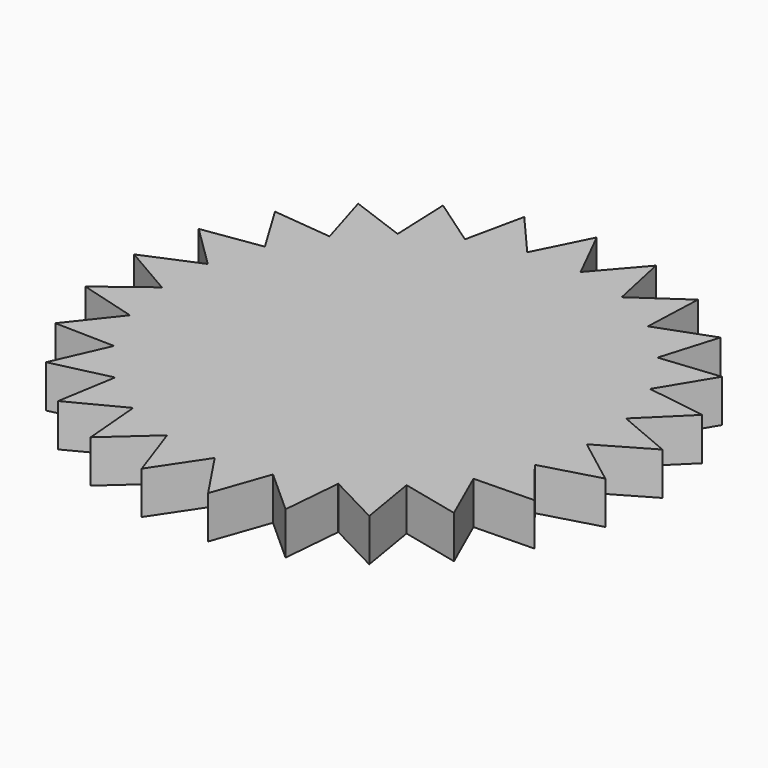
from build123d import *

# Parameters (mm, degrees)
F0_R            = 63.5
F1_DEPTH        = 6.35
F3_DEPTH        = 12.7
F3_COPIES_COUNT = 25


# Not quite as in the source:
# - a pattern or mirror of a feature is missing from the dataset's text; its kind, count and spacing are read off the source's solid


with BuildPart() as f1:
    # F0 (on Top) → F1 (new body, symmetric)
    with BuildSketch(Plane.XY):
        Circle(F0_R)
    extrude(amount=F1_DEPTH, both=True)

    # F2 (on face) → F3 (join, through all)
    with BuildSketch(Plane.XY.offset(6.35)):
        with BuildLine():
            Line((0, 78.9130567023), (-7.9355522703, 63.002198455))
            ThreePointArc((-7.9355522703, 63.002198455), (0, 63.5), (7.9355522703, 63.002198455))
            Line((7.9355522703, 63.002198455), (0, 78.9130567023))
        make_face()
    f3 = extrude(amount=-F3_DEPTH)

    # F3_copies: F3 ×25 about axis
    f3_copies_axis = Axis((0, 0, 0), (0, 0, 1))
    for i in range(1, F3_COPIES_COUNT):
        add(f3.rotate(f3_copies_axis, i * 360 / F3_COPIES_COUNT))


solid = f1.part
